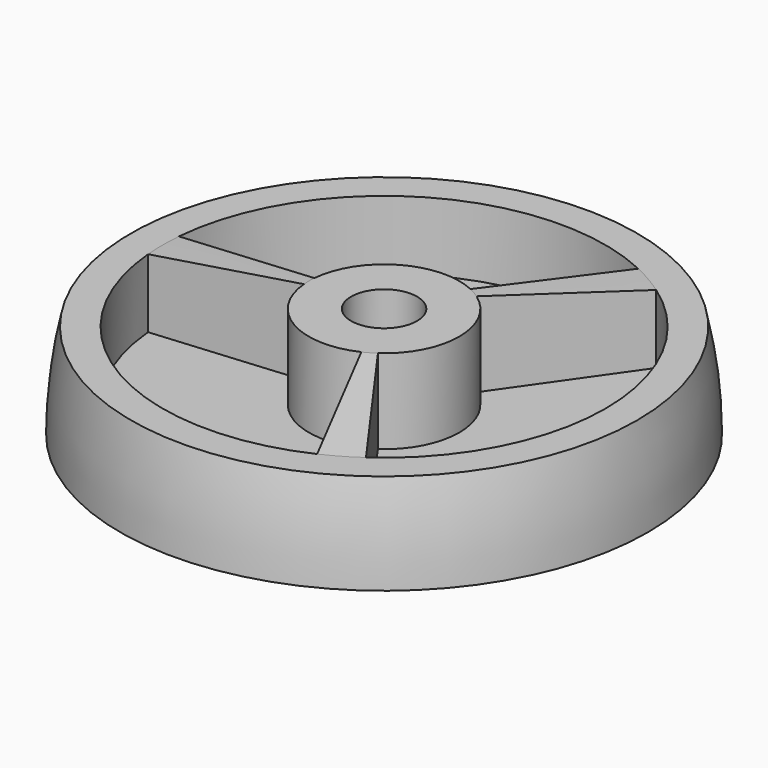
from build123d import *

# Parameters (mm, degrees)
F3_ANGLE_BACK   = 5
F3_ANGLE        = 10
F5_D            = 5.5
F5_COPIES_COUNT = 3
F8_ANGLE_BACK   = 5
F8_ANGLE        = 10


# Not quite as in the source:
# - a pattern or mirror of a feature is missing from the dataset's text; its kind, count and spacing are read off the source's solid


with BuildPart() as f1:
    # F0 (on Front) → F1 (revolve)
    with BuildSketch(Plane.XZ):
        with BuildLine():
            Line((41.9487010796, 5), (14.25, 5))
            Line((14.25, 5), (14.25, 21))
            Line((14.25, 21), (6.25, 21))
            Line((6.25, 21), (6.25, 0))
            Line((6.25, 0), (50, 0))
            ThreePointArc((50, 0), (49.4855209657, 9.058253519), (47.9487010796, 18))
            Line((47.9487010796, 18), (41.9487010796, 18))
            Line((41.9487010796, 18), (41.9487010796, 5))
        make_face()
    revolve(axis=Axis((0, 0, 8.5228504971), (0, 0, 1)))

    # F2 (on Front) → F3 (revolve)
    with BuildSketch(Plane.XZ, mode=Mode.PRIVATE) as f3_sk:
        Polygon((-14.25, 21), (-41.9487010796, 18), (-41.9487010796, 5), (-14.25, 5), align=None)
    f3 = revolve(f3_sk.sketch.rotate(Axis((0, 0, 5), (0, 0, 1)), -F3_ANGLE_BACK), axis=Axis((0, 0, 5), (0, 0, 1)), revolution_arc=F3_ANGLE)

    # F3_copies: F3 across plane
    add(f3.mirror(Plane(origin=(0, 0, 0), x_dir=(0.5, 0.8660254038, 0), z_dir=(0.8660254038, -0.5, 0))))

    # F5 (through all)
    with Locations(Plane.XY.offset(5)):
        with Locations((30, 0)):
            f5 = Hole(F5_D / 2)

    # F5_copies: F5 ×3 about axis
    f5_copies_axis = Axis((0, 0, 0), (0, 0, 1))
    for i in range(1, F5_COPIES_COUNT):
        add(f5.rotate(f5_copies_axis, i * 360 / F5_COPIES_COUNT), mode=Mode.SUBTRACT)

    # F7 (on face) → F8 (revolve)
    with BuildSketch(Plane(origin=(0, 0, 0), x_dir=(0.5, 0.8660254038, 0), z_dir=(0.8660254038, -0.5, 0)), mode=Mode.PRIVATE) as f8_sk:
        Polygon((14.25, 5), (41.9487010796, 5), (41.9487010796, 18), (14.25, 21), align=None)
    revolve(f8_sk.sketch.rotate(Axis((0, 0, 5), (0, 0, 1)), -F8_ANGLE_BACK), axis=Axis((0, 0, 5), (0, 0, 1)), revolution_arc=F8_ANGLE)


solid = f1.part
